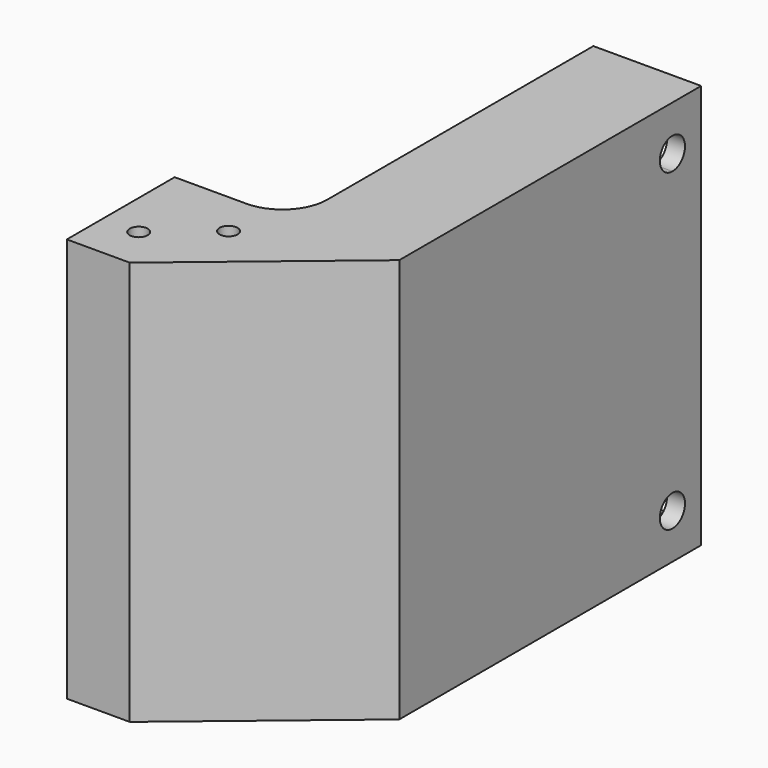
from build123d import *

# Parameters (mm, degrees)
F1_DEPTH  = 45
F3_DEPTH  = 2
F4_W      = 10
F4_H      = 42
F4_R      = 1
F5_DEPTH  = 2
F7_DEPTH  = 2
F8_R      = 5
F9_W      = 10
F9_H      = 10.2169760242
F10_DEPTH = 1
F11_W     = 9
F11_H     = 41
F12_DEPTH = 2
F16_DEPTH = 45.001


# Not quite as in the source:
# - a feature names something its author has since deleted; it is built from what else it names


with BuildPart() as f1:
    # F0 (on Top) → F1 (new body)
    with BuildSketch(Plane.XY):
        with BuildLine():
            Line((12, -42), (12, 0))
            Line((12, 0), (10, 0))
            Line((10, 0), (10, -42))
            Line((10, -42), (-4.5861525412, -54.7628834735))
            ThreePointArc((-4.5861525412, -54.7628834735), (-6.1200422145, -55.6805137201), (-7.8786755805, -56))
            Line((-7.8786755805, -56), (-13, -56))
            Line((-13, -56), (-13, -57))
            Line((-13, -57), (-6, -57))
            Line((-6, -57), (12, -42))
        make_face()
    extrude(amount=F1_DEPTH)

    # F2 (on face) → F3 (cut, through all)
    with BuildSketch(Plane(origin=(10, 0, 0), x_dir=(0, -1, 0), z_dir=(-1, 0, 0))):
        with BuildLine():
            ThreePointArc((4, 6.75), (2.7625631329, 3.7625631329), (5.75, 5))
            ThreePointArc((5.75, 5), (5.2374368671, 6.2374368671), (4, 6.75))
        make_face()
        with BuildLine():
            ThreePointArc((5.75, 40), (2.7625631329, 41.2374368671), (4, 38.25))
            ThreePointArc((4, 38.25), (5.2374368671, 38.7625631329), (5.75, 40))
        make_face()
    extrude(amount=-F3_DEPTH, mode=Mode.SUBTRACT)

    # F4 (on face) → F5 (join)
    with BuildSketch(Plane(origin=(0, 0, 0), x_dir=(1, 0, 0), z_dir=(0, 0, -1))):
        Polygon((10, 42), (12, 42), (0, 52), (0, 50.75), align=None)
        with Locations((5, 21)):
            Rectangle(F4_W, F4_H)
        Polygon((0, 42), (10, 42), (0, 50.75), align=None)
        with BuildLine():
            Line((0, 42), (0, 50.75))
            Line((0, 50.75), (-4.5861525412, 54.7628834735))
            ThreePointArc((-4.5861525412, 54.7628834735), (-6.1200422145, 55.6805137201), (-7.8786755805, 56))
            Line((-7.8786755805, 56), (-13, 56))
            Line((-13, 56), (-13, 42))
            Line((-13, 42), (0, 42))
        make_face()
        with Locations((-9, 52)):
            Circle(F4_R, mode=Mode.SUBTRACT)
        with Locations((-3, 47)):
            Circle(F4_R, mode=Mode.SUBTRACT)
        with Locations((-9, 52)):
            Circle(F4_R)
        with Locations((-3, 47)):
            Circle(F4_R)
    extrude(amount=-F5_DEPTH)

    # F6 (on face) → F7 (join)
    with BuildSketch(Plane.XY.offset(45)):
        Polygon((12, -42), (12, 0), (0, 0), (0, -42), (-13, -42), (-13, -57), (-6, -57), align=None)
    extrude(amount=-F7_DEPTH)

    # F8
    f8_edges = [f1.edges().sort_by_distance(p)[0] for p in [
        (0, -42, 44),
        (0, -42, 1),
    ]]
    fillet(f8_edges, radius=F8_R)

    # F9 (on face) → F10 (cut)
    with BuildSketch(Plane(origin=(0, 0, 43), x_dir=(1, 0, 0), z_dir=(0, 0, -1))):
        with Locations((5, 20.4747493975)):
            Rectangle(F9_W, F9_H)
    extrude(amount=-F10_DEPTH, mode=Mode.SUBTRACT)

    # F11 (on face) → F12 (join)
    with BuildSketch(Plane(origin=(-13, 0, 0), x_dir=(0, -1, 0), z_dir=(-1, 0, 0))):
        with Locations((46.5, 22.5)):
            Rectangle(F11_W, F11_H)
    extrude(amount=-F12_DEPTH)

    # F14 (on offset) → F15 (join, up to the next surface of F1)
    with BuildSketch(Plane.XZ.offset(42)):
        with BuildLine():
            ThreePointArc((-11, 43), (3.8492424049, 36.8492424049), (10, 22))
            Line((10, 22), (10, 43))
            Line((10, 43), (-11, 43))
        make_face()
    extrude(until=Until.NEXT)

    # F4 (on face) → F16 (cut, through all)
    with BuildSketch(Plane(origin=(0, 0, 0), x_dir=(1, 0, 0), z_dir=(0, 0, -1))):
        with Locations((-3, 47)):
            Circle(F4_R)
        with Locations((-9, 52)):
            Circle(F4_R)
    extrude(amount=-F16_DEPTH, mode=Mode.SUBTRACT)


solid = f1.part
